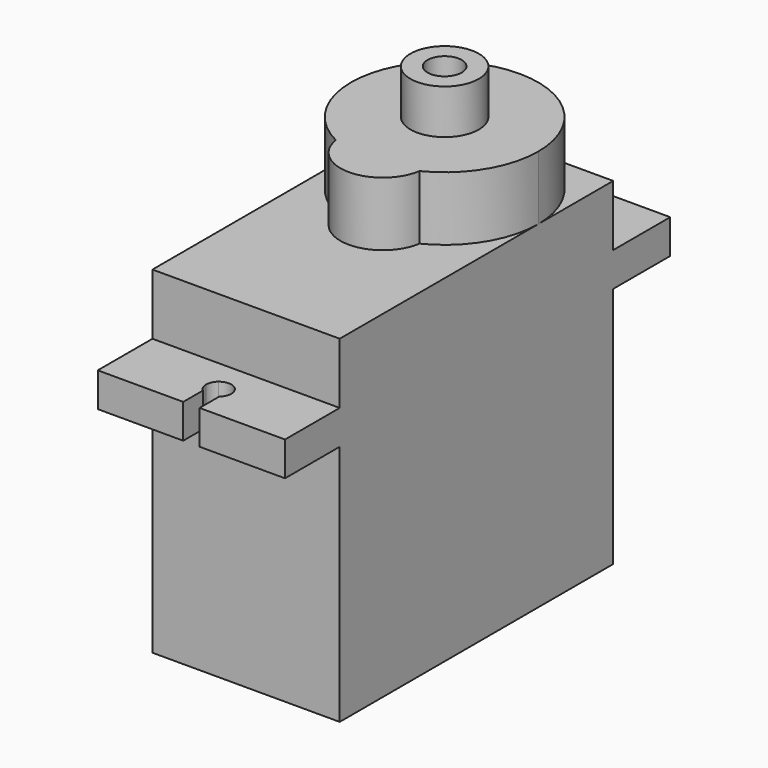
from build123d import *

# Parameters (mm, degrees)
F0_W     = 12.6
F0_H     = 23
F1_DEPTH = 16.3
F3_DEPTH = 2.3
F4_W     = 12.6
F4_H     = 23
F5_DEPTH = 4.1
F7_DEPTH = 4.3
F8_R     = 2.3
F8_R_2   = 1.15
F9_DEPTH = 3


with BuildPart() as f1:
    # F0 (on Top) → F1 (new body)
    with BuildSketch(Plane.XY):
        Rectangle(F0_W, F0_H)
    extrude(amount=F1_DEPTH)

    # F2 (on face) → F3 (join)
    with BuildSketch(Plane.XY.offset(16.3)):
        Polygon((-0.55, 11.5), (-6.3, 11.5), (-6.3, -11.5), (-0.55, -11.5), (0.55, -11.5), (6.3, -11.5), (6.3, 11.5), (0.55, 11.5), align=None)
        with BuildLine():
            Line((-6.3, 13.9), (-6.3, 11.5))
            Line((-6.3, 11.5), (-0.55, 11.5))
            Line((-0.55, 11.5), (-0.55, 13.2519259302))
            ThreePointArc((-0.55, 13.2519259302), (-0.771362431, 13.5429285786), (-0.85, 13.9))
            Line((-0.85, 13.9), (-6.3, 13.9))
        make_face()
        with BuildLine():
            Line((-6.3, 16.3), (-6.3, 13.9))
            Line((-6.3, 13.9), (-0.85, 13.9))
            ThreePointArc((-0.85, 13.9), (-0.771362431, 14.2570714214), (-0.55, 14.5480740698))
            Line((-0.55, 14.5480740698), (-0.55, 16.3))
            Line((-0.55, 16.3), (-6.3, 16.3))
        make_face()
        with BuildLine():
            Line((-0.55, 13.2519259302), (-0.55, 11.5))
            Line((-0.55, 11.5), (0.55, 11.5))
            Line((0.55, 11.5), (0.55, 13.2519259302))
            ThreePointArc((0.55, 13.2519259302), (0, 13.05), (-0.55, 13.2519259302))
        make_face()
        with BuildLine():
            Line((0.55, 13.2519259302), (0.55, 11.5))
            Line((0.55, 11.5), (6.3, 11.5))
            Line((6.3, 11.5), (6.3, 16.3))
            Line((6.3, 16.3), (0.55, 16.3))
            Line((0.55, 16.3), (0.55, 14.5480740698))
            ThreePointArc((0.55, 14.5480740698), (0.771362431, 14.2570714214), (0.85, 13.9))
            ThreePointArc((0.85, 13.9), (0.771362431, 13.5429285786), (0.55, 13.2519259302))
        make_face()
        with BuildLine():
            Line((6.3, -11.5), (0.55, -11.5))
            Line((0.55, -11.5), (0.55, -13.1519259302))
            ThreePointArc((0.55, -13.1519259302), (0.771362431, -13.4429285786), (0.85, -13.8))
            ThreePointArc((0.85, -13.8), (0.771362431, -14.1570714214), (0.55, -14.4480740698))
            Line((0.55, -14.4480740698), (0.55, -16.1))
            Line((0.55, -16.1), (6.3, -16.1))
            Line((6.3, -16.1), (6.3, -11.5))
        make_face()
        with BuildLine():
            Line((0.55, -11.5), (-0.55, -11.5))
            Line((-0.55, -11.5), (-0.55, -13.1519259302))
            ThreePointArc((-0.55, -13.1519259302), (0, -12.95), (0.55, -13.1519259302))
            Line((0.55, -13.1519259302), (0.55, -11.5))
        make_face()
        with BuildLine():
            Line((-0.55, -11.5), (-6.3, -11.5))
            Line((-6.3, -11.5), (-6.3, -13.8))
            Line((-6.3, -13.8), (-0.85, -13.8))
            ThreePointArc((-0.85, -13.8), (-0.771362431, -13.4429285786), (-0.55, -13.1519259302))
            Line((-0.55, -13.1519259302), (-0.55, -11.5))
        make_face()
        with BuildLine():
            Line((-0.85, -13.8), (-6.3, -13.8))
            Line((-6.3, -13.8), (-6.3, -16.1))
            Line((-6.3, -16.1), (-0.55, -16.1))
            Line((-0.55, -16.1), (-0.55, -14.4480740698))
            ThreePointArc((-0.55, -14.4480740698), (-0.771362431, -14.1570714214), (-0.85, -13.8))
        make_face()
    extrude(amount=F3_DEPTH)

    # F4 (on face) → F5 (join)
    with BuildSketch(Plane.XY.offset(18.6)):
        Rectangle(F4_W, F4_H)
    extrude(amount=F5_DEPTH)

    # F6 (on face) → F7 (join)
    with BuildSketch(Plane.XY.offset(22.7)):
        with BuildLine():
            ThreePointArc((6.3, 5.2), (4.4547727215, 9.6547727215), (0, 11.5))
            Line((0, 11.5), (0, 5.2))
            Line((0, 5.2), (0, 2.85))
            ThreePointArc((0, 2.85), (2.0152543264, 2.0152543264), (2.85, 0))
            ThreePointArc((2.85, 0), (2.8416264502, -0.2183096822), (2.8165550054, -0.4353365385))
            ThreePointArc((2.8165550054, -0.4353365385), (5.3588383319, 1.8874704933), (6.3, 5.2))
        make_face()
        with BuildLine():
            Line((0, 5.2), (0, 11.5))
            ThreePointArc((0, 11.5), (-4.4547727215, 9.6547727215), (-6.3, 5.2))
            ThreePointArc((-6.3, 5.2), (-5.3588383319, 1.8874704933), (-2.8165550054, -0.4353365385))
            ThreePointArc((-2.8165550054, -0.4353365385), (-2.1637015892, 1.8549650759), (0, 2.85))
            Line((0, 2.85), (0, 5.2))
        make_face()
        with BuildLine():
            ThreePointArc((2.85, 0), (2.0152543264, 2.0152543264), (0, 2.85))
            ThreePointArc((0, 2.85), (-2.1637015892, 1.8549650759), (-2.8165550054, -0.4353365385))
            ThreePointArc((-2.8165550054, -0.4353365385), (0, -1.1), (2.8165550054, -0.4353365385))
            ThreePointArc((2.8165550054, -0.4353365385), (2.8416264502, -0.2183096822), (2.85, 0))
        make_face()
        with BuildLine():
            ThreePointArc((-2.8165550054, -0.4353365385), (0, -2.85), (2.8165550054, -0.4353365385))
            ThreePointArc((2.8165550054, -0.4353365385), (0, -1.1), (-2.8165550054, -0.4353365385))
        make_face()
    extrude(amount=F7_DEPTH)

    # F8 (on face) → F9 (join)
    with BuildSketch(Plane.XY.offset(27)):
        with Locations((0, 5.2)):
            Circle(F8_R)
        with Locations((0, 5.2)):
            Circle(F8_R_2, mode=Mode.SUBTRACT)
    extrude(amount=F9_DEPTH)


solid = f1.part
